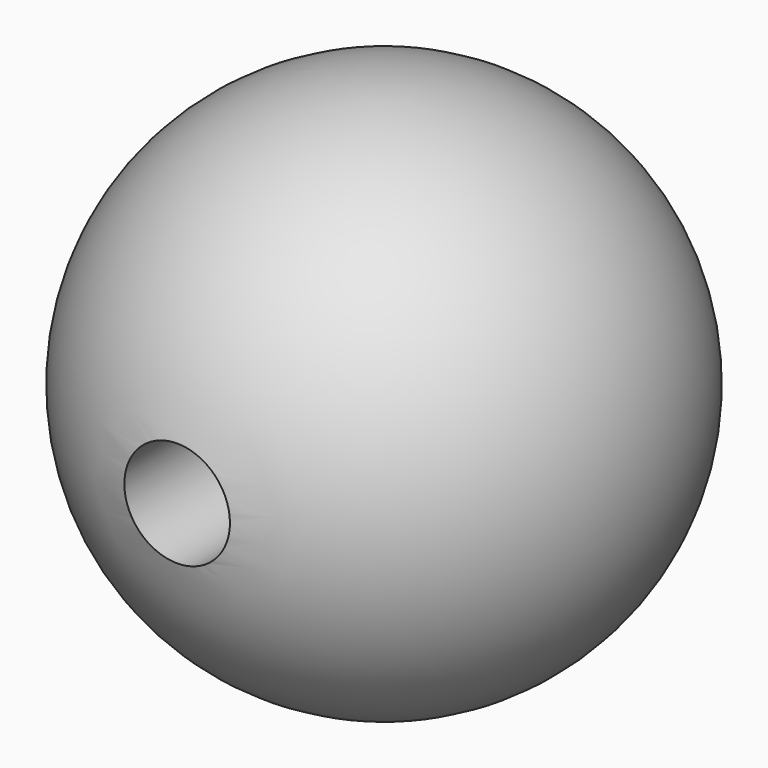
from build123d import *

# Parameters (mm, degrees)
F5_R          = 3.175
F6_DEPTH      = 50.8
F9_ANGLE      = 113.3
F11_TEXT_SIZE = 5.3138090556
F12_DEPTH     = 25.4
F13_ANGLE     = 108.8
F15_TEXT_SIZE = 3.53854266
F16_DEPTH     = 25.4


# Not quite as in the source:
# - a length typed as a fraction of an inch, garbled in the dataset ("3 / 203.2 mm" for 3/8 in), is restored
# - Text() gives the source's letters only with a copy of the font that has no kerning and outlines rounded to 1/6400 em; it was checked with that copy


with BuildPart() as f2:
    # F0 (on Front) → F2 (revolve)
    with BuildSketch(Plane.XZ):
        with BuildLine():
            Line((0, -15.875), (0, 15.875))
            ThreePointArc((0, 15.875), (-15.875, 0), (0, -15.875))
        make_face()
    revolve(axis=Axis((0, 0, 0), (0, 0, 1)))

    # F11 (on offset) → F12 (cut)
    with BuildSketch(Plane(origin=(0, 12.3073983122, -28.5774591555), x_dir=(1, 0, 0), z_dir=(0, 0.3955455026, -0.9184463813))):
        with Locations((-6.8843920308, 3.9062118158)):
            Text('113.3', F11_TEXT_SIZE, font='Open Sans', text_align=(TextAlign.LEFT, TextAlign.BOTTOM))
    extrude(amount=-F12_DEPTH, mode=Mode.SUBTRACT)

    # F15 (on offset) → F16 (cut)
    with BuildSketch(Plane(origin=(-27.0528305655, 12.3073983122, 9.2095347427), x_dir=(-0.3744428573, -0.9184463813, 0.1274707464), z_dir=(-0.8694465874, 0.3955455026, 0.2959837616))):
        with Locations((-4.2069517076, 4.0275598876)):
            Text('108.8', F15_TEXT_SIZE, font='Open Sans', text_align=(TextAlign.LEFT, TextAlign.BOTTOM))
    extrude(amount=-F16_DEPTH, mode=Mode.SUBTRACT)


with BuildPart() as f6:
    # F5 (on offset) → F6 (new body)
    with BuildSketch(Plane.XZ.offset(5.715)):
        Circle(F5_R)
    extrude(amount=F6_DEPTH)


with BuildPart() as f9_1:
    # F9: copy of F6
    add(f6.part.rotate(Axis((33.8576585054, 0, 0), (1, 0, 0)), F9_ANGLE))


with BuildPart() as f13_1:
    # F13: copy of F9_1
    add(f9_1.part.rotate(Axis((0, 32.2498939931, 0), (0, 1, 0)), F13_ANGLE))


with BuildPart() as f2_1:
    add(f2.part)

    # F17: cut F6, F13_1, F9_1
    add(f6.part, mode=Mode.SUBTRACT)
    add(f13_1.part, mode=Mode.SUBTRACT)
    add(f9_1.part, mode=Mode.SUBTRACT)


solid = f2_1.part
